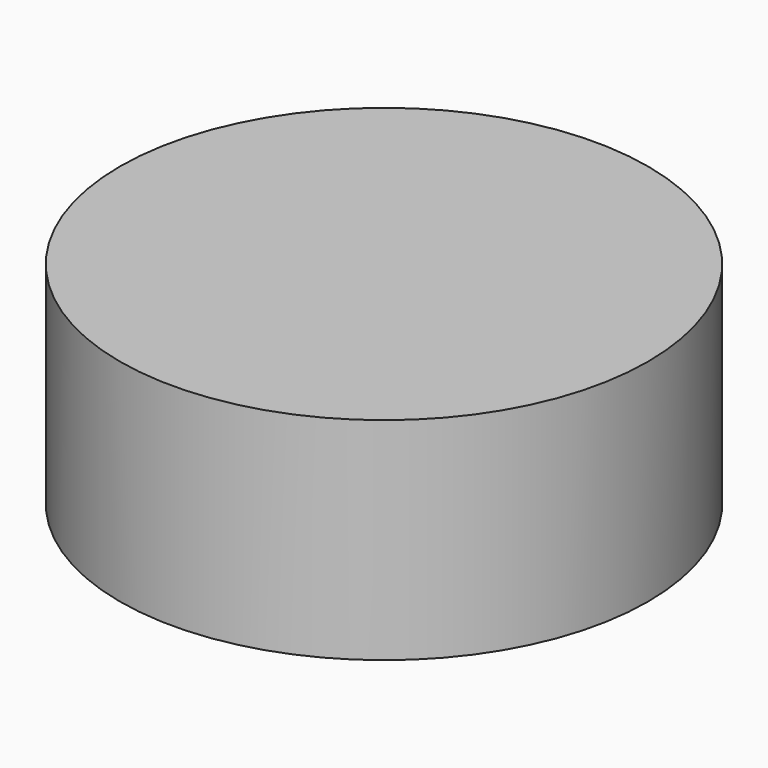
from build123d import *
from build123d import SkipClean  # not in build123d's __all__

# Parameters (mm, degrees)
F0_R     = 12.5
F1_DEPTH = 5
F2_DEPTH = 5.001
F3_DEPTH = 2.5


with BuildPart() as f1:
    # F0 (on Top) → F1 (new body, symmetric)
    with BuildSketch(Plane.XY):
        Circle(F0_R)
        with BuildLine():
            ThreePointArc((-2.8, -6.9577295147), (-4.1982139059, 6.2149014473), (7.5, 0))
            ThreePointArc((7.5, 0), (6.2149014473, -4.1982139059), (2.8, -6.9577295147))
            Line((2.8, -6.9577295147), (2.8, -10))
            Line((2.8, -10), (0, -10))
            Line((0, -10), (-2.8, -10))
            Line((-2.8, -10), (-2.8, -6.9577295147))
        make_face(mode=Mode.SUBTRACT)
        with BuildLine():
            ThreePointArc((2.8, -6.9577295147), (6.2149014473, -4.1982139059), (7.5, 0))
            ThreePointArc((7.5, 0), (-4.1982139059, 6.2149014473), (-2.8, -6.9577295147))
            ThreePointArc((-2.8, -6.9577295147), (0, -7.5), (2.8, -6.9577295147))
        make_face()
        with BuildLine():
            ThreePointArc((2.8, -6.9577295147), (0, -7.5), (-2.8, -6.9577295147))
            Line((-2.8, -6.9577295147), (-2.8, -10))
            Line((-2.8, -10), (0, -10))
            Line((0, -10), (2.8, -10))
            Line((2.8, -10), (2.8, -6.9577295147))
        make_face()
    extrude(amount=F1_DEPTH, both=True)

    # F0 (on Top) → F2 (cut, through all)
    with BuildSketch(Plane.XY):
        with BuildLine():
            ThreePointArc((2.8, -6.9577295147), (0, -7.5), (-2.8, -6.9577295147))
            Line((-2.8, -6.9577295147), (-2.8, -10))
            Line((-2.8, -10), (0, -10))
            Line((0, -10), (2.8, -10))
            Line((2.8, -10), (2.8, -6.9577295147))
        make_face()
        with BuildLine():
            ThreePointArc((2.8, -6.9577295147), (6.2149014473, -4.1982139059), (7.5, 0))
            ThreePointArc((7.5, 0), (-4.1982139059, 6.2149014473), (-2.8, -6.9577295147))
            ThreePointArc((-2.8, -6.9577295147), (0, -7.5), (2.8, -6.9577295147))
        make_face()
    extrude(amount=-F2_DEPTH, mode=Mode.SUBTRACT)

    # F0 (on Top) → F3 (join)
    with BuildSketch(Plane.XY):
        with BuildLine():
            ThreePointArc((2.8, -6.9577295147), (0, -7.5), (-2.8, -6.9577295147))
            Line((-2.8, -6.9577295147), (-2.8, -10))
            Line((-2.8, -10), (0, -10))
            Line((0, -10), (2.8, -10))
            Line((2.8, -10), (2.8, -6.9577295147))
        make_face()
    with SkipClean():  # cleaning this boolean's faces spoils the solid; the shape is the same uncleaned
        extrude(amount=-F3_DEPTH)


solid = f1.part
